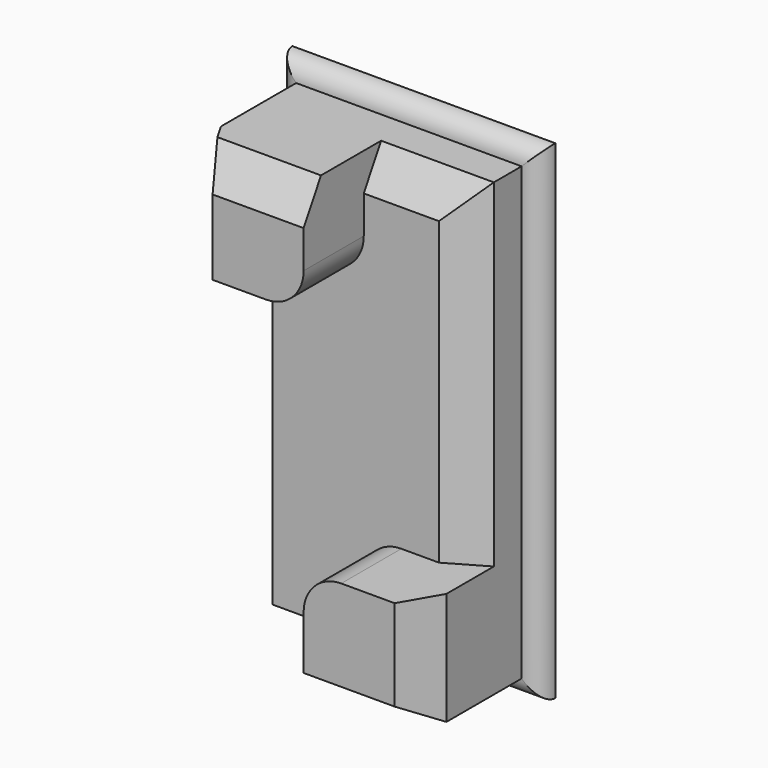
from build123d import *

# Parameters (mm, degrees)
F0_W        = 88.8999989152
F0_H        = 165.0999989152
F1_DEPTH    = 6.35
F2_DEPTH    = 25.4
F3_DEPTH    = 50.8
F4_C1_SIZE2 = 7.3323484187
F4_C1_SIZE  = 12.7
F4_C2_SIZE2 = 7.3323484187
F4_C2_SIZE  = 12.7
F4_C3_SIZE2 = 7.3323484187
F4_C3_SIZE  = 12.7
F4_C4_SIZE2 = 12.7
F4_C4_SIZE  = 7.3323484187
F4_C5_SIZE2 = 7.3323484187
F4_C5_SIZE  = 12.7
F4_C6_SIZE2 = 7.3323484187
F4_C6_SIZE  = 12.7
F4_C7_SIZE2 = 12.7
F4_C7_SIZE  = 7.3323484187
F4_C8_SIZE2 = 12.7
F4_C8_SIZE  = 7.3323484187
F5_R        = 6.34999


# Not quite as in the source:
# - a fillet or chamfer is up to 0.001 mm smaller than in the source, because OpenCascade refuses the exact size


with BuildPart() as f1:
    # F0 (on Front) → F1 (new body)
    with BuildSketch(Plane.XZ):
        with Locations((-44.4499994576, -82.5499994576)):
            Rectangle(F0_W, F0_H)
        Polygon((-82.5499994576, -44.4499994576), (-82.5499994576, -6.3499994576), (-44.4499994576, -6.3499994576), (-6.3499994576, -6.3499994576), (-6.3499994576, -120.6499994576), (-6.3499994576, -158.7499994576), (-44.4499994576, -158.7499994576), (-82.5499994576, -158.7499994576), align=None, mode=Mode.SUBTRACT)
    extrude(amount=F1_DEPTH)

    # F0 (on Front) → F2 (join)
    with BuildSketch(Plane.XZ):
        with BuildLine():
            Line((-57.1499994576, -44.4499994576), (-82.5499994576, -44.4499994576))
            Line((-82.5499994576, -44.4499994576), (-82.5499994576, -158.7499994576))
            Line((-82.5499994576, -158.7499994576), (-44.4499994576, -158.7499994576))
            Line((-44.4499994576, -158.7499994576), (-44.4499994576, -133.3499994576))
            ThreePointArc((-44.4499994576, -133.3499994576), (-40.7302555787, -124.3697433365), (-31.7499994576, -120.6499994576))
            Line((-31.7499994576, -120.6499994576), (-6.3499994576, -120.6499994576))
            Line((-6.3499994576, -120.6499994576), (-6.3499994576, -6.3499994576))
            Line((-6.3499994576, -6.3499994576), (-44.4499994576, -6.3499994576))
            Line((-44.4499994576, -6.3499994576), (-44.4499994576, -31.7499994576))
            ThreePointArc((-44.4499994576, -31.7499994576), (-48.1697433365, -40.7302555787), (-57.1499994576, -44.4499994576))
        make_face()
    extrude(amount=F2_DEPTH)

    # F0 (on Front) → F3 (join)
    with BuildSketch(Plane.XZ):
        with BuildLine():
            Line((-44.4499994576, -6.3499994576), (-82.5499994576, -6.3499994576))
            Line((-82.5499994576, -6.3499994576), (-82.5499994576, -44.4499994576))
            Line((-82.5499994576, -44.4499994576), (-57.1499994576, -44.4499994576))
            ThreePointArc((-57.1499994576, -44.4499994576), (-48.1697433365, -40.7302555787), (-44.4499994576, -31.7499994576))
            Line((-44.4499994576, -31.7499994576), (-44.4499994576, -6.3499994576))
        make_face()
        with BuildLine():
            Line((-44.4499994576, -133.3499994576), (-44.4499994576, -158.7499994576))
            Line((-44.4499994576, -158.7499994576), (-6.3499994576, -158.7499994576))
            Line((-6.3499994576, -158.7499994576), (-6.3499994576, -120.6499994576))
            Line((-6.3499994576, -120.6499994576), (-31.7499994576, -120.6499994576))
            ThreePointArc((-31.7499994576, -120.6499994576), (-40.7302555787, -124.3697433365), (-44.4499994576, -133.3499994576))
        make_face()
    extrude(amount=F3_DEPTH)

    # F4: chamfer of 12.7 x 7.3323484187 on 8 edges, made by hand

    # F4_c1
    f4_c1_edges = [f1.edges().sort_by_distance(p)[0] for p in [
        (-63.4999994576, -25.4, -158.7499994576),
    ]]
    f4_c1_side = f1.faces().sort_by_distance((-63.4999994576, -25.2533530316, -158.7499994576))[0]
    chamfer(f4_c1_edges, length=F4_C1_SIZE, length2=F4_C1_SIZE2, reference=f4_c1_side)

    # F4_c2
    f4_c2_edges = [f1.edges().sort_by_distance(p)[0] for p in [
        (-25.3999994576, -50.8, -158.7499994576),
    ]]
    f4_c2_side = f1.faces().sort_by_distance((-25.3999994576, -50.6533530316, -158.7499994576))[0]
    chamfer(f4_c2_edges, length=F4_C2_SIZE, length2=F4_C2_SIZE2, reference=f4_c2_side)

    # F4_c3
    f4_c3_edges = [f1.edges().sort_by_distance(p)[0] for p in [
        (-6.3499994576, -50.8, -136.0338252482),
    ]]
    f4_c3_side = f1.faces().sort_by_distance((-6.3499994576, -50.6533530316, -136.0338252482))[0]
    chamfer(f4_c3_edges, length=F4_C3_SIZE, length2=F4_C3_SIZE2, reference=f4_c3_side)

    # F4_c4
    f4_c4_edges = [f1.edges().sort_by_distance(p)[0] for p in [
        (-82.5499994576, -25.4, -97.9338252482),
    ]]
    f4_c4_side = f1.faces().sort_by_distance((-82.4033524892, -25.4, -97.9338252482))[0]
    chamfer(f4_c4_edges, length=F4_C4_SIZE, length2=F4_C4_SIZE2, reference=f4_c4_side)

    # F4_c5
    f4_c5_edges = [f1.edges().sort_by_distance(p)[0] for p in [
        (-6.3499994576, -25.4, -63.4999994576),
    ]]
    f4_c5_side = f1.faces().sort_by_distance((-6.496646426, -25.4, -63.4999994576))[0]
    chamfer(f4_c5_edges, length=F4_C5_SIZE, length2=F4_C5_SIZE2, reference=f4_c5_side)

    # F4_c6
    f4_c6_edges = [f1.edges().sort_by_distance(p)[0] for p in [
        (-31.7499994576, -25.4, -6.3499994576),
    ]]
    f4_c6_side = f1.faces().sort_by_distance((-31.7499994576, -25.4, -6.496646426))[0]
    chamfer(f4_c6_edges, length=F4_C6_SIZE, length2=F4_C6_SIZE2, reference=f4_c6_side)

    # F4_c7
    f4_c7_edges = [f1.edges().sort_by_distance(p)[0] for p in [
        (-63.4999994576, -50.8, -6.3499994576),
    ]]
    f4_c7_side = f1.faces().sort_by_distance((-63.4999994576, -50.6533530316, -6.3499994576))[0]
    chamfer(f4_c7_edges, length=F4_C7_SIZE, length2=F4_C7_SIZE2, reference=f4_c7_side)

    # F4_c8
    f4_c8_edges = [f1.edges().sort_by_distance(p)[0] for p in [
        (-82.5499994576, -50.8, -31.7499994576),
    ]]
    f4_c8_side = f1.faces().sort_by_distance((-82.4033524892, -50.8, -31.7499994576))[0]
    chamfer(f4_c8_edges, length=F4_C8_SIZE, length2=F4_C8_SIZE2, reference=f4_c8_side)

    # F5 (radius 6.35 in the source; OpenCascade refuses exactly that, so slightly less here)
    f5_edges = [f1.edges().sort_by_distance(p)[0] for p in [
        (-44.449999, -6.35, 0),
        (-88.899999, -6.35, -82.549999),
        (0, -6.35, -82.549999),
        (-44.449999, -6.35, -165.099999),
    ]]
    fillet(f5_edges, radius=F5_R)


solid = f1.part
